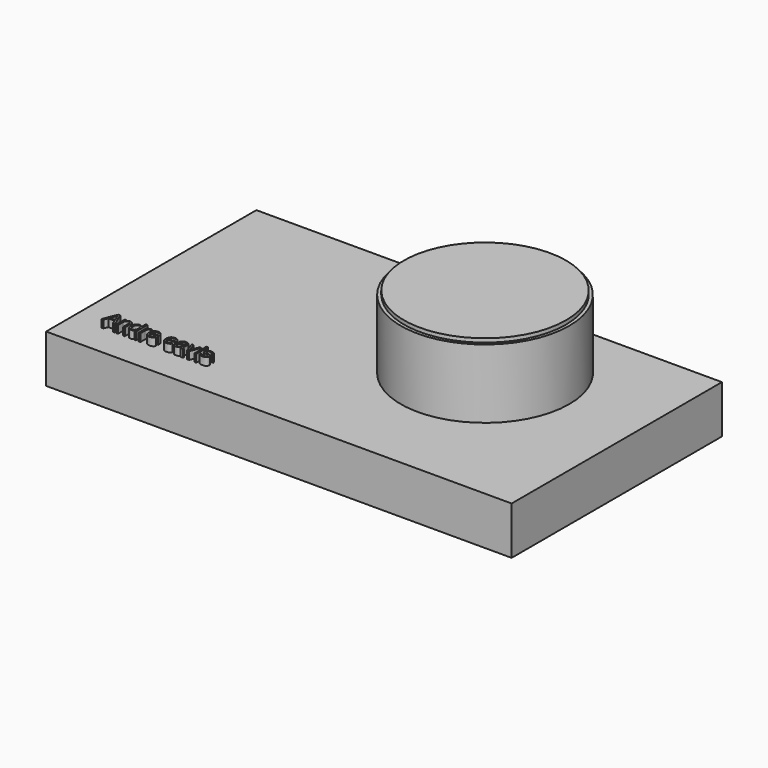
from build123d import *

# Parameters (mm, degrees)
F0_W          = 243.0755496025
F0_H          = 137.2521519661
F1_DEPTH      = 25
F2_W          = 19.89787817
F2_H          = 12.8333196044
F3_DEPTH      = 23
F4_R          = 44.004
F5_DEPTH      = 36
F6_T          = -2.5
F8_DEPTH      = 11
F9_R          = 42.3068115043
F10_DEPTH     = 2
F11_TEXT_SIZE = 10.4983544184
F12_DEPTH     = 4


# Not quite as in the source:
# - Text() gives the source's letters only with a copy of the font that has no kerning and outlines rounded to 1/6400 em; it was checked with that copy


with BuildPart() as f1:
    # F0 (on Top) → F1 (new body)
    with BuildSketch(Plane.XY):
        Rectangle(F0_W, F0_H)
    extrude(amount=F1_DEPTH)

    # F2 (on face) → F3 (join)
    with BuildSketch(Plane.XY.offset(25)):
        with Locations((30.7846702635, 75.0427357852)):
            Rectangle(F2_W, F2_H)
    extrude(amount=-F3_DEPTH)

    # F4 (on face) → F5 (join)
    with BuildSketch(Plane.XY.offset(25)):
        with Locations((41.1087423563, 14.5418569446)):
            Circle(F4_R)
    extrude(amount=F5_DEPTH)

    # F6
    f6_openings = [f1.faces().sort_by_distance(p)[0] for p in [
        (41.108742, 14.541857, 61),
    ]]
    offset(amount=F6_T, openings=f6_openings, kind=Kind.INTERSECTION)

    # F7 (on face) → F8 (join)
    with BuildSketch(Plane.XY.offset(2.5)):
        Polygon((50.6358208242, 39.0701229929), (38.8013937825, 24.9222011019), (42.3332363608, 20.7357742222), (46.154653101, 20.1092112404), (60.440765197, 17.7668472428), (63.0321608494, 29.980480862), align=None)
    extrude(amount=F8_DEPTH)

    # F9 (on face) → F10 (join)
    with BuildSketch(Plane.XY.offset(61)):
        with Locations((41.1087423563, 14.5418569446)):
            Circle(F9_R)
    extrude(amount=F10_DEPTH)

    # F11 (on face) → F12 (join)
    with BuildSketch(Plane.XY.offset(25)):
        with Locations((-106.0223057866, -51.8657714128)):
            Text('Andre eavis', F11_TEXT_SIZE, font='Arimo', text_align=(TextAlign.LEFT, TextAlign.BOTTOM))
    extrude(amount=F12_DEPTH)


solid = f1.part
